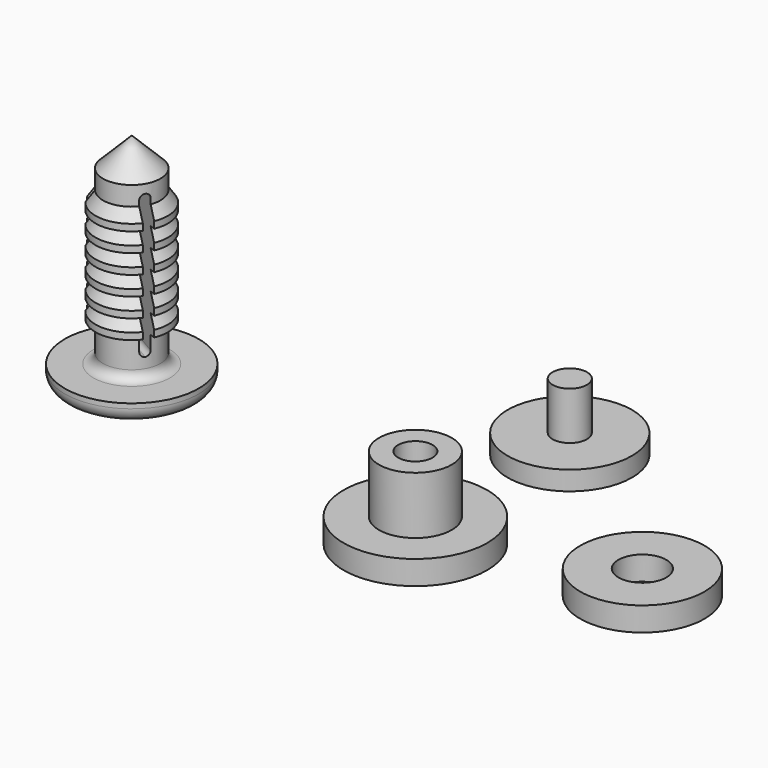
from build123d import *

# Parameters (mm, degrees)
F0_R      = 7.5
F1_DEPTH  = 2.5
F2_R      = 3.8
F3_DEPTH  = 6
F4_T      = -2
F5_R      = 6.5
F6_DEPTH  = 2
F7_R      = 1.8
F8_DEPTH  = 5
F9_R      = 6.5
F9_R_2    = 2.5
F10_DEPTH = 2.5
F15_DEPTH = 15
F16_R     = 1
F17_R     = 1.5
F18_R     = 0.4999


# Not quite as in the source:
# - a fillet or chamfer is up to 0.001 mm smaller than in the source, because OpenCascade refuses the exact size
# - a feature names something its author has since deleted; it is built from what else it names


with BuildPart() as f1:
    # F0 (on Top) → F1 (new body)
    with BuildSketch(Plane.XY):
        Circle(F0_R)
    extrude(amount=F1_DEPTH)

    # F2 (on face) → F3 (join)
    with BuildSketch(Plane.XY.offset(2.5)):
        Circle(F2_R)
    extrude(amount=F3_DEPTH)

    # F4
    f4_openings = [f1.faces().sort_by_distance(p)[0] for p in [
        (0, 0, 8.5),
    ]]
    offset(amount=F4_T, openings=f4_openings, kind=Kind.INTERSECTION)


with BuildPart() as f6:
    # F5 (on Top) → F6 (new body)
    with BuildSketch(Plane.XY):
        with Locations((0, 20.1621446759)):
            Circle(F5_R)
    extrude(amount=F6_DEPTH)

    # F7 (on face) → F8 (join)
    with BuildSketch(Plane.XY.offset(2)):
        with Locations((0, 20.1621446759)):
            Circle(F7_R)
    extrude(amount=F8_DEPTH)


with BuildPart() as f10:
    # F9 (on Top) → F10 (new body)
    with BuildSketch(Plane.XY):
        with Locations((20.2099084854, 4.3817702681)):
            Circle(F9_R)
        with Locations((20.2099084854, 4.3817702681)):
            Circle(F9_R_2, mode=Mode.SUBTRACT)
    extrude(amount=F10_DEPTH)


with BuildPart() as f12:
    # F11 (on Front) → F12 (revolve)
    with BuildSketch(Plane.XZ):
        Polygon((-36.6300484105, 4.9155716072), (-29.6300484105, 4.9155716072), (-29.6300484105, 27.9155716072), (-32.6300484105, 24.9155716072), (-32.6300484105, 22.9155716072), (-33.4178946129, 21.7544901494), (-33.4178946129, 21.0544901494), (-32.6300484105, 20.9155716072), (-33.4178946129, 19.7544901494), (-33.4178946129, 19.0544901494), (-32.6300484105, 18.9155716072), (-33.4178946129, 17.7544901494), (-33.4178946129, 17.0544901494), (-32.6300484105, 16.9155716072), (-33.4178946129, 15.7544901494), (-33.4178946129, 15.0544901494), (-32.6300484105, 14.9155716072), (-33.4178946129, 13.7544901494), (-33.4178946129, 13.0544901494), (-32.6300484105, 12.9155716072), (-33.4178946129, 11.7544901494), (-33.4178946129, 11.0544901494), (-32.6300484105, 10.9155716072), (-32.6300484105, 6.9155716072), (-36.6300484105, 6.9155716072), align=None)
    revolve(axis=Axis((-29.6300484105, 0, 16.4155716072), (0, 0, 1)))

    # F14 (on offset) → F15 (cut)
    with BuildSketch(Plane.XY.offset(24)):
        Polygon((-30.1300484105, 0.2886751346), (-30.1300484105, 0), (-29.6300484105, 0), (-29.8800484105, 0.4330127019), align=None)
        Polygon((-29.6300484105, 0), (-30.1300484105, 0), (-30.1300484105, 0.2886751346), (-40.2723532559, -5.5669872981), (-39.7723532559, -6.4330127019), (-29.6300484105, -0.5773502692), (-29.8800484105, -0.4330127019), align=None)
        Polygon((-29.3800484105, 0.4330127019), (-29.6300484105, 0), (-29.1300484105, 0), (-29.1300484105, 0.2886751346), align=None)
        Polygon((-29.1300484105, 0), (-29.6300484105, 0), (-29.3800484105, -0.4330127019), (-29.6300484105, -0.5773502692), (-19.487743565, -6.4330127019), (-18.987743565, -5.5669872981), (-29.1300484105, 0.2886751346), align=None)
        Polygon((-29.8800484105, 0.4330127019), (-29.6300484105, 0), (-29.3800484105, 0.4330127019), (-29.1300484105, 0.2886751346), (-29.1300484105, 12), (-30.1300484105, 12), (-30.1300484105, 0.2886751346), align=None)
        Polygon((-29.3800484105, -0.4330127019), (-29.6300484105, 0), (-29.8800484105, -0.4330127019), (-29.6300484105, -0.5773502692), align=None)
    extrude(amount=-F15_DEPTH, mode=Mode.SUBTRACT)

    # F16
    f16_edges = [f12.edges().sort_by_distance(p)[0] for p in [
        (-26.630048, 0, 6.915572),
    ]]
    fillet(f16_edges, radius=F16_R)

    # F17
    f17_edges = [f12.edges().sort_by_distance(p)[0] for p in [
        (-22.630048, 0, 4.915572),
    ]]
    fillet(f17_edges, radius=F17_R)

    # F18 (radius 0.5 in the source; OpenCascade refuses exactly that, so slightly less here)
    f18_edges = [f12.edges().sort_by_distance(p)[0] for p in [
        (-29.130048, 1.623358, 9),
        (-30.130048, 1.623358, 9),
        (-27.97418, -0.378666, 9),
        (-28.47418, -1.244691, 9),
        (-31.285917, -0.378666, 9),
        (-30.785917, -1.244691, 9),
        (-29.130048, 1.623358, 24),
        (-31.285917, -0.378666, 24),
        (-27.97418, -0.378666, 24),
        (-30.785917, -1.244691, 24),
        (-30.130048, 1.623358, 24),
        (-28.47418, -1.244691, 24),
    ]]
    fillet(f18_edges, radius=F18_R)


solid = Compound([f1.part, f6.part, f10.part, f12.part])
